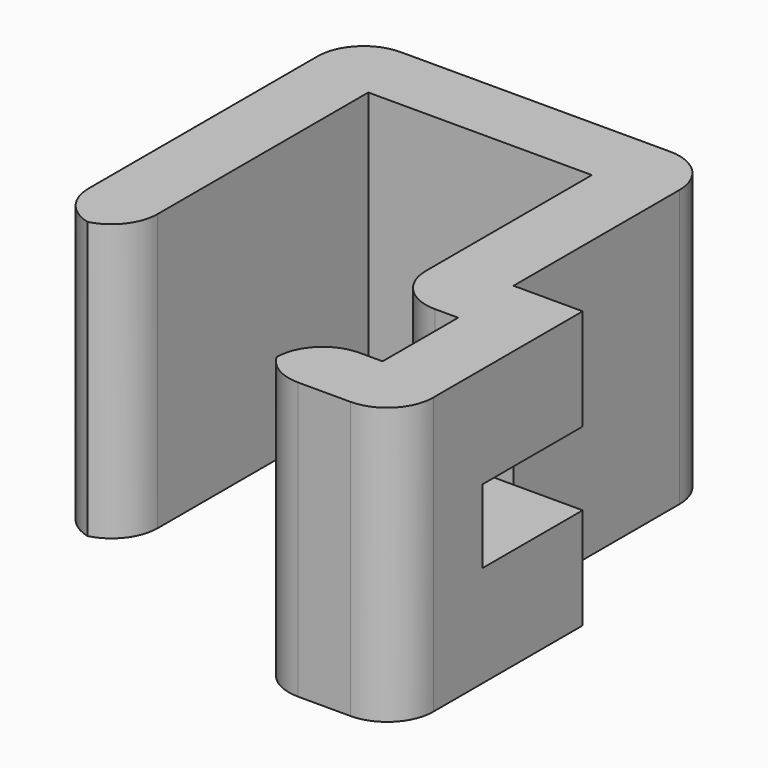
from build123d import *

# Parameters (mm, degrees)
F1_DEPTH    = 15.24
F3_DEPTH    = 9.779
F4_R        = 2.54
F5_T1_DEPTH = 27.94
F5_T3_DEPTH = 26.2385226281
F5_T5_DEPTH = 18.288
F5_T7_DEPTH = 18.288


# Not quite as in the source:
# - a fillet or chamfer that OpenCascade refuses, or shapes differently, is made with other operations: its cross-section is extruded or revolved along the edge and cut away or added


with BuildPart() as f1:
    # F0 (on Top) → F1 (new body)
    with BuildSketch(Plane.XY):
        Polygon((0, 20.8534), (0, 0), (3.81, 0), (3.81, 17.0434), (16.129, 17.0434), (16.129, 3.0734), (19.939, 3.0734), (19.939, -2.1336), (16.129, -2.1336), (16.129, -5.9436), (23.749, -5.9436), (23.749, 6.8834), (19.939, 6.8834), (19.939, 20.8534), align=None)
    extrude(amount=F1_DEPTH)

    # F2 (on face) → F3 (cut)
    with BuildSketch(Plane.YZ.offset(23.749)):
        Polygon((0, 5.588), (6.8834, 5.588), (6.8834, 7.62), (6.8834, 9.652), (0, 9.652), (0, 7.62), align=None)
    extrude(amount=-F3_DEPTH, mode=Mode.SUBTRACT)

    # F4
    f4_edges = [f1.edges().sort_by_distance(p)[0] for p in [
        (0, 20.8534, 7.62),
        (19.939, 20.8534, 7.62),
        (23.749, -5.9436, 7.62),
        (16.129, -2.1336, 7.62),
    ]]
    fillet(f4_edges, radius=F4_R)

    # F5: fillet of radius 2.54 on 5 edges, made by hand

    # F5_s2 → F5_t1 (cut)
    with BuildSketch(Plane.XY.offset(-6.35)):
        with BuildLine():
            ThreePointArc((0, 2.54), (0.7439487758, 0.7439487758), (2.54, 0))
            Line((2.54, 0), (2.54, -0.0508))
            Line((2.54, -0.0508), (-0.0508, -0.0508))
            Line((-0.0508, -0.0508), (-0.0508, 2.54))
            Line((-0.0508, 2.54), (0, 2.54))
        make_face()
        with BuildLine():
            ThreePointArc((1.27, 0), (3.0660512242, 0.7439487758), (3.81, 2.54))
            Line((3.81, 2.54), (3.8608, 2.54))
            Line((3.8608, 2.54), (3.8608, -0.0508))
            Line((3.8608, -0.0508), (1.27, -0.0508))
            Line((1.27, -0.0508), (1.27, 0))
        make_face()
    extrude(amount=F5_T1_DEPTH, mode=Mode.SUBTRACT)

    # F5_s4 → F5_t3 (cut)
    with BuildSketch(Plane.XY.offset(-5.499261314)):
        with BuildLine():
            ThreePointArc((18.3287045256, -5.9436), (17.0587045256, -5.6033045256), (16.129, -4.6736))
            Line((16.129, -4.6736), (16.0850059095, -4.699))
            ThreePointArc((16.0850059095, -4.699), (16.0782, -5.3086), (16.0782, -5.9436))
            Line((16.0782, -5.9436), (16.129, -5.9944))
            Line((16.129, -5.9944), (18.3287045256, -5.9944))
            Line((18.3287045256, -5.9944), (18.3287045256, -5.9436))
        make_face()
    extrude(amount=F5_T3_DEPTH, mode=Mode.SUBTRACT)

    # F5_s6 → F5_t5 (cut)
    with BuildSketch(Plane.XY.offset(-6.35)):
        with BuildLine():
            ThreePointArc((16.129, 5.6134), (16.8729487758, 3.8173487758), (18.669, 3.0734))
            Line((18.669, 3.0734), (18.669, 3.0226))
            Line((18.669, 3.0226), (16.0782, 3.0226))
            Line((16.0782, 3.0226), (16.0782, 5.6134))
            Line((16.0782, 5.6134), (16.129, 5.6134))
        make_face()
    extrude(amount=F5_T5_DEPTH, mode=Mode.SUBTRACT)

    # F5_s8 → F5_t7 (cut)
    with BuildSketch(Plane.XY.offset(3.302)):
        with BuildLine():
            ThreePointArc((16.129, 5.6134), (16.8729487758, 3.8173487758), (18.669, 3.0734))
            Line((18.669, 3.0734), (18.669, 3.0226))
            Line((18.669, 3.0226), (16.0782, 3.0226))
            Line((16.0782, 3.0226), (16.0782, 5.6134))
            Line((16.0782, 5.6134), (16.129, 5.6134))
        make_face()
    extrude(amount=F5_T7_DEPTH, mode=Mode.SUBTRACT)


solid = f1.part
